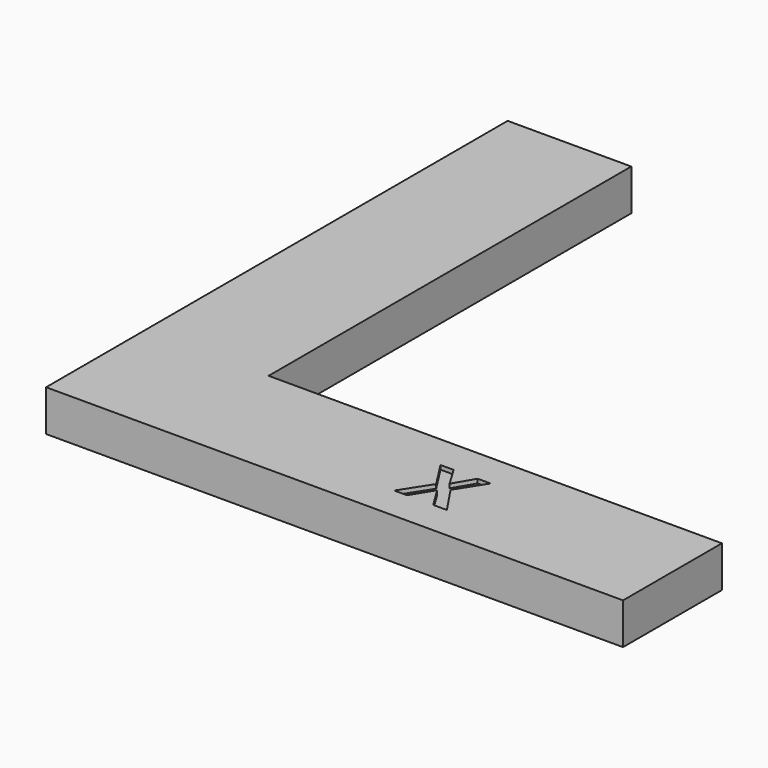
from build123d import *

# Parameters (mm, degrees)
F1_DEPTH     = 5
F2_TEXT_SIZE = 9.5644748079
F3_DEPTH     = 0.5


# Not quite as in the source:
# - Text() gives the source's letters only with a copy of the font that has no kerning and outlines rounded to 1/6400 em; it was checked with that copy


with BuildPart() as f1:
    # F0 (on Top) → F1 (new body)
    with BuildSketch(Plane.XY):
        Polygon((0, 0), (0, 54.9999960124), (-15, 54.9999960124), (-15, -15), (55, -15), (55, 0), align=None)
    extrude(amount=F1_DEPTH)

    # F2 (on face) → F3 (cut)
    with BuildSketch(Plane.XY.offset(5)):
        with Locations((24, -10.9432109308)):
            Text('X', F2_TEXT_SIZE, font='Open Sans', font_style=FontStyle.BOLD, text_align=(TextAlign.LEFT, TextAlign.BOTTOM))
    extrude(amount=-F3_DEPTH, mode=Mode.SUBTRACT)


solid = f1.part
